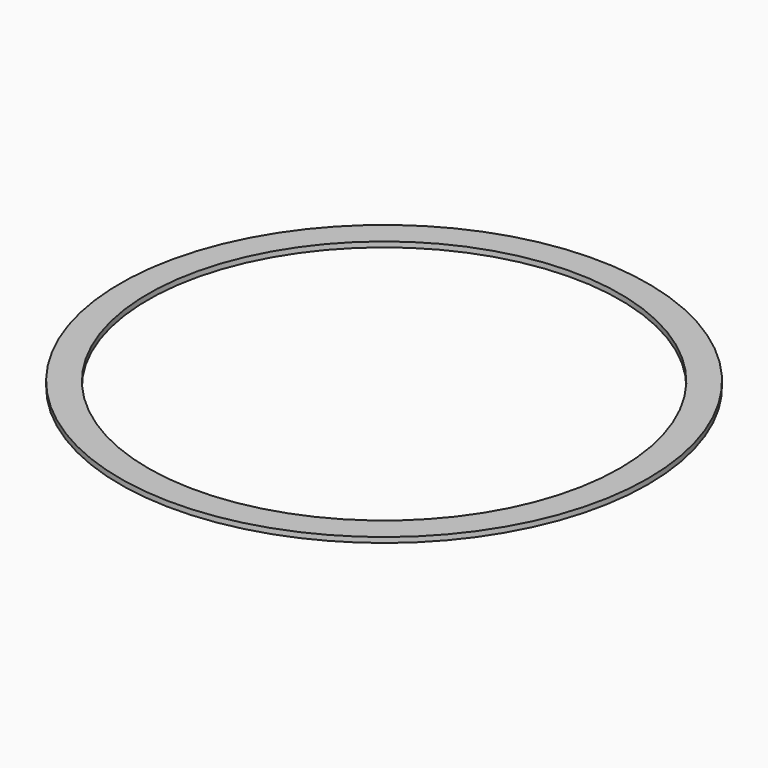
from build123d import *

# Parameters (mm, degrees)
F0_R     = 240.05794
F0_R_2   = 214.65794
F1_DEPTH = 4.7625


# Not quite as in the source:
# - a length typed as a fraction of an inch, garbled in the dataset ("3 / 203.2 mm" for 3/8 in), is restored


with BuildPart() as f1:
    # F0 (on Top) → F1 (new body)
    with BuildSketch(Plane.XY):
        Circle(F0_R)
        Circle(F0_R_2, mode=Mode.SUBTRACT)
    extrude(amount=F1_DEPTH)


solid = f1.part
